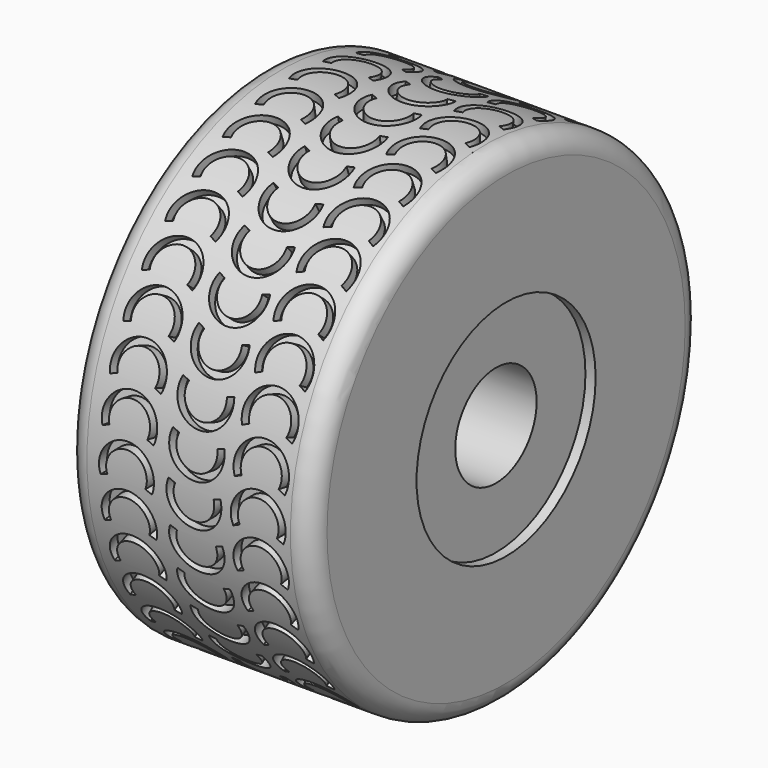
from build123d import *

# Parameters (mm, degrees)
F5_DEPTH        = 0.5
F5_COPIES_COUNT = 36


# Not quite as in the source:
# - a pattern or mirror of a feature is missing from the dataset's text; its kind, count and spacing are read off the source's solid


with BuildPart() as f1:
    # F0 (on Top) → F1 (revolve)
    with BuildSketch(Plane.XY):
        with BuildLine():
            Line((0, 11), (0, 5.5))
            Line((0, 5.5), (0.5, 5.5))
            Line((0.5, 5.5), (0.5, 2.5))
            Line((0.5, 2.5), (11.5, 2.5))
            Line((11.5, 2.5), (11.5, 5.5))
            Line((11.5, 5.5), (12, 5.5))
            Line((12, 5.5), (12, 11))
            ThreePointArc((12, 11), (11.7071067812, 11.7071067812), (11, 12))
            Line((11, 12), (1, 12))
            ThreePointArc((1, 12), (0.2928932188, 11.7071067812), (0, 11))
        make_face()
    revolve(axis=Axis((6, 0, 0), (1, 0, 0)))

    # F4 (on offset) → F5 (cut)
    with BuildSketch(Plane.XZ.offset(12)):
        with BuildLine():
            ThreePointArc((1.9998655231, -0.3137630712), (2.971248986, 1.0175340106), (3.8666006481, -0.3660422082))
            Line((3.8666006481, -0.3660422082), (4.1897718669, -0.5004310595))
            ThreePointArc((4.1897718669, -0.5004310595), (2.9810471231, 1.3673968359), (1.6696794481, -0.4298542245))
            Line((1.6696794481, -0.4298542245), (1.9998655231, -0.3137630712))
        make_face()
        with BuildLine():
            ThreePointArc((7.2179597057, 0.2932616019), (6.2059614461, -0.9807905213), (5.3280517087, 0.3891086658))
            Line((5.3280517087, 0.3891086658), (5.0030557635, 0.5190226205))
            ThreePointArc((5.0030557635, 0.5190226205), (6.188233909, -1.3303412822), (7.5544315594, 0.3896290841))
            Line((7.5544315594, 0.3896290841), (7.2179597057, 0.2932616019))
        make_face()
        with BuildLine():
            ThreePointArc((8.5035090171, -0.3857328266), (9.4293158308, 1.0178665621), (10.3243139775, -0.4055756804))
            Line((10.3243139775, -0.4055756804), (10.6413773488, -0.553801247))
            ThreePointArc((10.6413773488, -0.553801247), (9.4331298508, 1.3678457804), (8.1832906523, -0.5270133944))
            Line((8.1832906523, -0.5270133944), (8.5035090171, -0.3857328266))
        make_face()
    f5 = extrude(amount=-F5_DEPTH, mode=Mode.SUBTRACT)

    # F5_copies: F5 ×36 about axis
    f5_copies_axis = Axis((0, 0, 0), (1, 0, 0))
    for i in range(1, F5_COPIES_COUNT):
        add(f5.rotate(f5_copies_axis, i * 360 / F5_COPIES_COUNT), mode=Mode.SUBTRACT)


solid = f1.part
